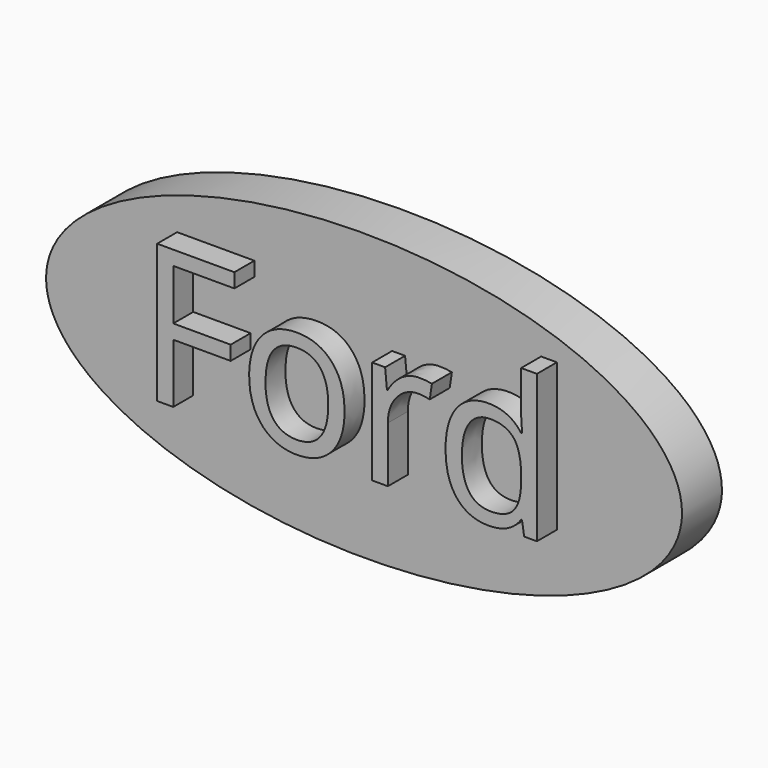
from build123d import *

# Parameters (mm, degrees)
F1_DEPTH     = 6.35
F2_TEXT_SIZE = 24.6868779262
F3_DEPTH     = 3.175


# Not quite as in the source:
# - Text() gives the source's letters only with a copy of the font that has no kerning and outlines rounded to 1/6400 em; it was checked with that copy


with BuildPart() as f1:
    # F0 (on Front) → F1 (new body)
    with BuildSketch(Plane.XZ):
        with BuildLine():
            add(Edge.make_bspline(
                [(13.3994221687, 23.0624638498), (13.3994221687, 54.5423246965), (-47.2844950855, 38.8023942731), (-107.9684123397, 23.0624638498), (-47.2844950855, 7.3225334264), (13.3994221687, -8.4173969969), (13.3994221687, 23.0624638498)],
                knots=[0, 0, 0, 2.0943951024, 2.0943951024, 4.1887902048, 4.1887902048, 6.2831853072, 6.2831853072, 6.2831853072], degree=2, weights=[1, 0.5, 1, 0.5, 1, 0.5, 1]))
        make_face()
    extrude(amount=F1_DEPTH)

    # F2 (on face) → F3 (join)
    with BuildSketch(Plane.XZ.offset(6.35)):
        with Locations((-53.2594269607, 16.0023327917)):
            Text('Ford', F2_TEXT_SIZE, font='Open Sans', text_align=(TextAlign.LEFT, TextAlign.BOTTOM))
    extrude(amount=F3_DEPTH)


solid = f1.part
